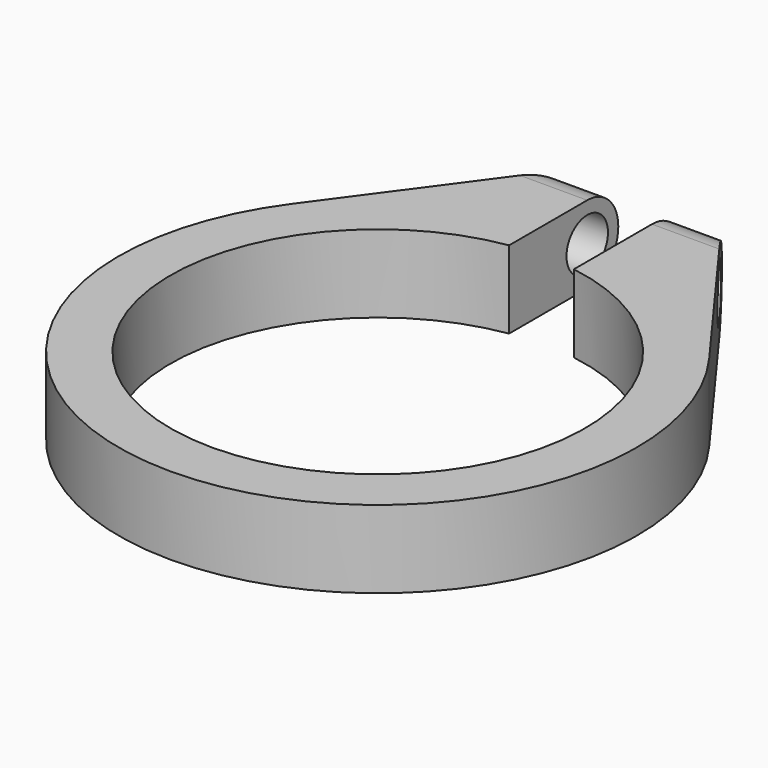
from build123d import *

# Parameters (mm, degrees)
F1_DEPTH      = 7.62
F2_R          = 2.54
F3_DEPTH      = 25.4
F3_DEPTH_BACK = 25.4
F4_R          = 3.81
F5_R          = 3.80999


# Not quite as in the source:
# - a fillet or chamfer is up to 0.001 mm smaller than in the source, because OpenCascade refuses the exact size


with BuildPart() as f1:
    # F0 (on Top) → F1 (new body)
    with BuildSketch(Plane.XY):
        with BuildLine():
            ThreePointArc((3.175, 20.0704203992), (0, -20.32), (-3.175, 20.0704203992))
            Line((-3.175, 20.0704203992), (-3.175, 33.4507006653))
            Line((-3.175, 33.4507006653), (-6.985, 33.4507006653))
            Line((-6.985, 33.4507006653), (-20.4920611043, 15.0078456714))
            ThreePointArc((-20.4920611043, 15.0078456714), (0, -25.4), (20.4920611043, 15.0078456714))
            Line((20.4920611043, 15.0078456714), (6.985, 33.4507006653))
            Line((6.985, 33.4507006653), (3.175, 33.4507006653))
            Line((3.175, 33.4507006653), (3.175, 20.0704203992))
        make_face()
    extrude(amount=F1_DEPTH)

    # F2 (on face) → F3 (cut, two sides)
    with BuildSketch(Plane.YZ.offset(-3.175)) as f3_sk:
        with Locations((29.6407006653, 3.81)):
            Circle(F2_R)
    extrude(amount=F3_DEPTH, mode=Mode.SUBTRACT)
    extrude(f3_sk.sketch, amount=-F3_DEPTH_BACK, mode=Mode.SUBTRACT)

    # F4
    f4_edges = [f1.edges().sort_by_distance(p)[0] for p in [
        (-5.08, 33.450701, 0),
        (5.08, 33.450701, 0),
    ]]
    fillet(f4_edges, radius=F4_R)

    # F5 (radius 3.81 in the source; OpenCascade refuses exactly that, so slightly less here)
    f5_edges = [f1.edges().sort_by_distance(p)[0] for p in [
        (-5.08, 33.450701, 7.62),
        (5.08, 33.450701, 7.62),
    ]]
    fillet(f5_edges, radius=F5_R)


solid = f1.part
